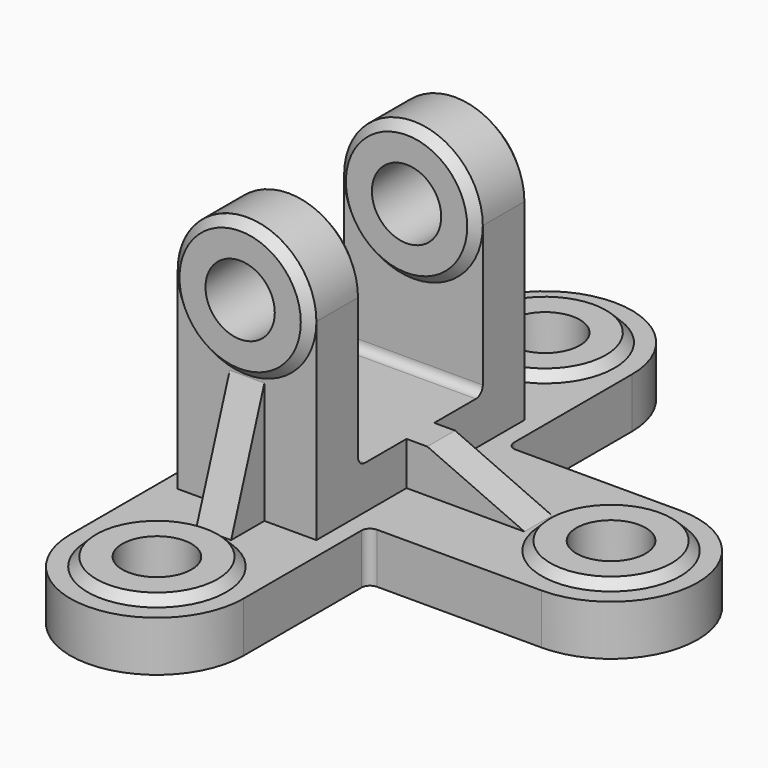
from build123d import *
from build123d import SkipClean  # not in build123d's __all__

# Parameters (mm, degrees)
F1_DEPTH  = 14.5
F3_DEPTH  = 20
F5_DEPTH  = 5
F7_DEPTH  = 5
F9_DEPTH  = 2.5
F10_DEPTH = 15
F12_DEPTH = 2.5
F14_SIZE  = 2.49999
F16_DEPTH = 15
F18_DEPTH = 2.5
F22_R     = 20
F23_DEPTH = 2.5
F24_SIZE  = 2.49999
F25_R     = 10
F26_DEPTH = 17.001
F27_R     = 10
F28_DEPTH = 17.001
F29_R     = 10
F30_DEPTH = 135.001
F31_R     = 10
F32_DEPTH = 75.501
F33_R     = 10
F34_DEPTH = 90.001
F35_R     = 2.5


# Not quite as in the source:
# - a fillet or chamfer that OpenCascade refuses, or shapes differently, is made with other operations: its cross-section is extruded or revolved along the edge and cut away or added
# - a fillet or chamfer is up to 0.001 mm smaller than in the source, because OpenCascade refuses the exact size
# - a feature of the source that left no trace in its solid (it failed there, or was rolled back) is left out
# - a pattern or mirror of a feature is missing from the dataset's text; its kind, count and spacing are read off the source's solid


with BuildPart() as f1:
    # F0 (on Top) → F1 (new body)
    with BuildSketch(Plane.XY):
        with BuildLine():
            ThreePointArc((25, 70), (0, 95), (-25, 70))
            Line((-25, 70), (-25, -70))
            ThreePointArc((-25, -70), (0, -95), (25, -70))
            Line((25, -70), (25, -25))
            Line((25, -25), (75, -25))
            ThreePointArc((75, -25), (100, 0), (75, 25))
            Line((75, 25), (25, 25))
            Line((25, 25), (25, 70))
        make_face()
    extrude(amount=F1_DEPTH)

    # F2 (on Right) → F3 (join, symmetric)
    with BuildSketch(Plane.YZ):
        Polygon((-37.5, 70), (-37.5, 0), (37.5, 0), (37.5, 70), (22.5, 70), (22.5, 27), (-22.5, 27), (-22.5, 70), align=None)
    extrude(amount=F3_DEPTH, both=True)

    # F4 (on Right) → F5 (join, symmetric)
    with BuildSketch(Plane.YZ):
        Polygon((-37.5, 49.5), (-49.5, 14.5), (-37.5, 14.5), align=None)
        Polygon((37.5, 49.5), (37.5, 14.5), (49.5, 14.5), align=None)
    extrude(amount=F5_DEPTH, both=True)

    # F6 (on Front) → F7 (join, symmetric)
    with BuildSketch(Plane.XZ):
        Polygon((26, 27), (20, 27), (20, 14.5), (54, 14.5), align=None)
    extrude(amount=F7_DEPTH, both=True)

    # F8 (on face) → F9 (join)
    with BuildSketch(Plane.XZ.offset(37.5)):
        with BuildLine():
            ThreePointArc((-20, 70), (0, 50), (20, 70))
            Line((20, 70), (-20, 70))
        make_face()
        with BuildLine():
            Line((-20, 70), (20, 70))
            ThreePointArc((20, 70), (0, 90), (-20, 70))
        make_face()
    extrude(amount=F9_DEPTH)

    # F10 (add): a face of the model
    f10_faces = [f1.faces().sort_by_distance(p)[0] for p in [
        (0, -37.5, 78.4882636316),
    ]]
    extrude(f10_faces, amount=F10_DEPTH)

    # F11 (on face) → F12 (join)
    with BuildSketch(Plane(origin=(0, -22.5, 0), x_dir=(-1, 0, 0), z_dir=(0, 1, 0))):
        with BuildLine():
            ThreePointArc((-20, 70), (0, 50), (20, 70))
            ThreePointArc((20, 70), (0, 90), (-20, 70))
        make_face()
    f12 = extrude(amount=F12_DEPTH)

    # F12_copies: F12 across plane
    add(f12.mirror(Plane.ZX), clean=False)

    # F13: chamfer of 2.5 on 1 edges, made by hand

    # F13_s1 → F13_t2 (revolve, cut)
    with BuildSketch(Plane.XY.offset(70)):
        Polygon((20, -22.5), (17.5, -20), (20, -20), align=None)
    revolve(axis=Axis((0, -20, 70), (0, -1, 0)), mode=Mode.SUBTRACT)

    # F14 (size 2.5 in the source; OpenCascade refuses exactly that, so slightly less here)
    f14_edges = [f1.edges().sort_by_distance(p)[0] for p in [
        (-20, -40, 70),
    ]]
    chamfer(f14_edges, length=F14_SIZE)

    # F15 (on face) → F16 (join)
    with BuildSketch(Plane(origin=(0, 37.5, 0), x_dir=(-1, 0, 0), z_dir=(0, 1, 0))):
        with BuildLine():
            ThreePointArc((-20, 70), (0, 50), (20, 70))
            Line((20, 70), (-20, 70))
        make_face()
        with BuildLine():
            Line((-20, 70), (20, 70))
            ThreePointArc((20, 70), (0, 90), (-20, 70))
        make_face()
    extrude(amount=-F16_DEPTH)

    # F17 (on face) → F18 (join)
    with BuildSketch(Plane(origin=(0, 37.5, 0), x_dir=(-1, 0, 0), z_dir=(0, 1, 0))):
        with BuildLine():
            ThreePointArc((-20, 70), (0, 50), (20, 70))
            ThreePointArc((20, 70), (0, 90), (-20, 70))
        make_face()
    with SkipClean():  # cleaning this boolean's faces spoils the solid; the shape is the same uncleaned
        extrude(amount=F18_DEPTH)

    # F21: chamfer of 2.5 on 2 edges, made by hand

    # F21_s1 → F21_t2 (revolve, cut)
    with BuildSketch(Plane.XY.offset(70)):
        Polygon((20, 37.5), (17.5, 40), (20, 40), align=None)
    revolve(axis=Axis((0, 40, 70), (0, -1, 0)), mode=Mode.SUBTRACT)

    # F21_s3 → F21_t4 (revolve, cut)
    with BuildSketch(Plane.XY.offset(70)):
        Polygon((20, 22.5), (17.5, 20), (20, 20), align=None)
    revolve(axis=Axis((0, 20, 70), (0, -1, 0)), mode=Mode.SUBTRACT)

    # F22 (on face) → F23 (join)
    with BuildSketch(Plane.XY.offset(14.5)):
        with Locations((0, 70)):
            Circle(F22_R)
        with Locations((75, 0)):
            Circle(F22_R)
        with Locations((0, -70)):
            Circle(F22_R)
    extrude(amount=F23_DEPTH)

    # F24 (size 2.5 in the source; OpenCascade refuses exactly that, so slightly less here)
    f24_edges = [f1.edges().sort_by_distance(p)[0] for p in [
        (-20, 70, 17),
        (55, 0, 17),
        (-20, -70, 17),
    ]]
    chamfer(f24_edges, length=F24_SIZE)

    # F25 (on face) → F26 (cut, through all)
    with BuildSketch(Plane.XY.offset(17)):
        with Locations((0, 70)):
            Circle(F25_R)
    extrude(amount=-F26_DEPTH, mode=Mode.SUBTRACT)

    # F27 (on face) → F28 (cut, through all)
    with BuildSketch(Plane.XY.offset(17)):
        with Locations((75, 0)):
            Circle(F27_R)
    extrude(amount=-F28_DEPTH, mode=Mode.SUBTRACT)

    # F29 (on face) → F30 (cut, through all)
    with BuildSketch(Plane.XZ.offset(40)):
        with Locations((0, 70)):
            Circle(F29_R)
    extrude(amount=-F30_DEPTH, mode=Mode.SUBTRACT)

    # F31 (on face) → F32 (cut, through all)
    with BuildSketch(Plane.XY.offset(14.5)):
        with Locations((0, -70)):
            Circle(F31_R)
    extrude(amount=F32_DEPTH, mode=Mode.SUBTRACT)

    # F33 (on face) → F34 (cut, through all)
    with BuildSketch(Plane(origin=(0, 0, 0), x_dir=(1, 0, 0), z_dir=(0, 0, -1))):
        with Locations((0, 70)):
            Circle(F33_R)
    extrude(amount=-F34_DEPTH, mode=Mode.SUBTRACT)

    # F35
    f35_edges = [f1.edges().sort_by_distance(p)[0] for p in [
        (0, 22.5, 27),
        (0, -22.5, 27),
        (25, 25, 7.25),
        (25, -25, 7.25),
    ]]
    fillet(f35_edges, radius=F35_R)


solid = f1.part
